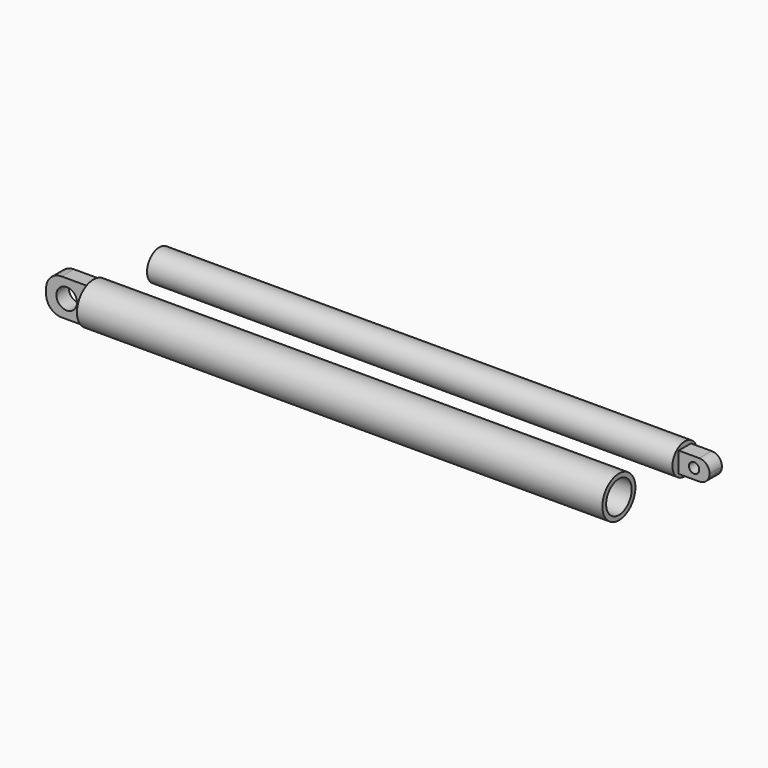
from build123d import *

# Parameters (mm, degrees)
F0_R      = 25.4
F1_DEPTH  = 647.7
F0_R_2    = 19.05
F2_R      = 19.685
F3_DEPTH  = 612.14
F4_W      = 19.05
F4_H      = 44.45
F5_DEPTH  = 50.8
F6_R      = 12.7
F7_DEPTH  = 130.176
F8_R      = 19.05
F9_W      = 19.05
F9_H      = 25.4
F10_DEPTH = 38.1
F11_R     = 6.35
F12_DEPTH = 136.526
F13_R     = 12.69999


# Not quite as in the source:
# - a fillet or chamfer is up to 0.001 mm smaller than in the source, because OpenCascade refuses the exact size


with BuildPart() as f1:
    # F0 (on Right) → F1 (new body)
    with BuildSketch(Plane.YZ):
        with Locations((-47.1377661452, 18.6495184898)):
            Circle(F0_R)
    extrude(amount=F1_DEPTH)

    # F2 (on face) → F3 (cut)
    with BuildSketch(Plane.YZ.offset(647.7)):
        with Locations((-47.1377661452, 18.6495184898)):
            Circle(F2_R)
    extrude(amount=-F3_DEPTH, mode=Mode.SUBTRACT)

    # F4 (on face) → F5 (join)
    with BuildSketch(Plane(origin=(0, 0, 0), x_dir=(0, -1, 0), z_dir=(-1, 0, 0))):
        with Locations((47.1377661452, 18.6495184898)):
            Rectangle(F4_W, F4_H)
    extrude(amount=F5_DEPTH)

    # F6 (on face) → F7 (cut, through all)
    with BuildSketch(Plane.XZ.offset(56.6627661452)):
        with Locations((-25.4, 18.6495184898)):
            Circle(F6_R)
    extrude(amount=-F7_DEPTH, mode=Mode.SUBTRACT)

    # F8
    f8_edges = [f1.edges().sort_by_distance(p)[0] for p in [
        (-50.8, -47.137766, 40.874518),
        (-50.8, -47.137766, -3.575482),
    ]]
    fillet(f8_edges, radius=F8_R)


with BuildPart() as f1b:
    # F0 (on Right) → F1, piece 2 (new body)
    with BuildSketch(Plane.YZ):
        with Locations((54.4622338548, 18.6495184898)):
            Circle(F0_R_2)
    extrude(amount=F1_DEPTH)

    # F9 (on face) → F10 (join)
    with BuildSketch(Plane.YZ.offset(647.7)):
        with Locations((54.4622338548, 18.8497592449)):
            Rectangle(F9_W, F9_H)
    extrude(amount=F10_DEPTH)

    # F11 (on face) → F12 (cut, through all)
    with BuildSketch(Plane(origin=(0, 63.9872338548, 0), x_dir=(-1, 0, 0), z_dir=(0, 1, 0))):
        with Locations((-666.75, 18.8497592449)):
            Circle(F11_R)
    extrude(amount=-F12_DEPTH, mode=Mode.SUBTRACT)

    # F13 (radius 12.7 in the source; OpenCascade refuses exactly that, so slightly less here)
    f13_edges = [f1b.edges().sort_by_distance(p)[0] for p in [
        (685.8, 54.462234, 31.549759),
        (685.8, 54.462234, 6.149759),
    ]]
    fillet(f13_edges, radius=F13_R)


solid = Compound([f1.part, f1b.part])
